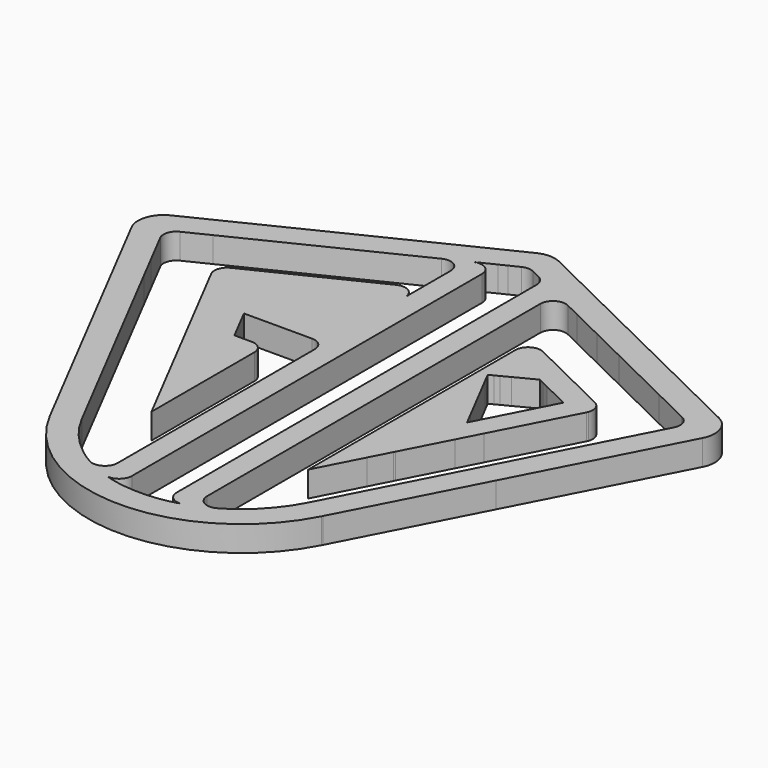
from build123d import *

# Parameters (mm, degrees)
F1_DEPTH = 1


# Not quite as in the source:
# - ends of sketch curves that miss each other by under 0.0002 mm in the source are joined
# - a feature names something its author has since deleted; it is built from what else it names


with BuildPart() as f1:
    # F0 (on Top) → F1 (new body)
    with BuildSketch(Plane.XY):
        with BuildLine():
            ThreePointArc((-11.7378467649, 8.9264858588), (-12.17732, 9.0282301738), (-12.6167932351, 8.9264858588))
            Line((-12.6167932351, 8.9264858588), (-22.9360292278, 3.8777807945))
            ThreePointArc((-22.9360292278, 3.8777807945), (-23.4460487393, 3.2933140895), (-23.3847383062, 2.5200338931))
            Line((-23.3847383062, 2.5200338931), (-17.5064138811, -8.8425854586))
            ThreePointArc((-17.5064138811, -8.8425854586), (-12.17732, -12.0856381601), (-6.8482261189, -8.8425854586))
            Line((-6.8482261189, -8.8425854586), (-6.8193229677, -8.786716561))
            Line((-6.8193229677, -8.786716561), (-4.1547760271, -3.6362297146))
            Line((-4.1547760271, -3.6362297146), (-0.9699016938, 2.5200338931))
            ThreePointArc((-0.9699016938, 2.5200338931), (-0.9085912607, 3.2933140895), (-1.4186107722, 3.8777807945))
            Line((-1.4186107722, 3.8777807945), (-11.7378467649, 8.9264858588))
        make_face()
        with BuildLine():
            ThreePointArc((-13.9352129405, -9.9781848161), (-14.1856518225, -10.4114506102), (-14.6860899339, -10.4106900001))
            ThreePointArc((-14.6860899339, -10.4106900001), (-14.9764347702, -10.2286994079), (-15.253632646, -10.0272495698))
            ThreePointArc((-15.253632646, -10.0272495698), (-16.0247836651, -9.2789159973), (-16.6182315676, -8.3830942422))
            Line((-16.6182315676, -8.3830942422), (-21.0987998739, 0.2777057515))
            Line((-21.0987998739, 0.2777057515), (-21.5773427489, 1.202714332))
            Line((-21.5773427489, 1.202714332), (-22.2616031934, 2.5253686134))
            ThreePointArc((-22.2616031934, 2.5253686134), (-22.29225841, 2.9120087116), (-22.0372486542, 3.2042420641))
            Line((-22.0372486542, 3.2042420641), (-21.0987998739, 3.6633798445))
            Line((-21.0987998739, 3.6633798445), (-14.6549495581, 6.8160453855))
            ThreePointArc((-14.6549495581, 6.8160453855), (-14.1705134022, 6.7911040048), (-13.9352129405, 6.366917543))
            Line((-13.9352129405, 6.366917543), (-13.9352129405, 4.1403800065))
            ThreePointArc((-13.9352129405, 4.1403800065), (-14.1705134022, 4.5645664683), (-14.6549495581, 4.589507849))
            Line((-14.6549495581, 4.589507849), (-15.253632646, 4.2966010544))
            Line((-15.253632646, 4.2966010544), (-18.9906600384, 2.4682535744))
            Line((-18.9906600384, 2.4682535744), (-18.5866887981, 1.687389658))
            Line((-18.5866887981, 1.687389658), (-16.9010777379, 2.5120779491))
            Line((-16.9010777379, 2.5120779491), (-14.6549495581, 3.6110002651))
            ThreePointArc((-14.6549495581, 3.6110002651), (-14.1705134022, 3.5860588844), (-13.9352129405, 3.1618724226))
            Line((-13.9352129405, 3.1618724226), (-13.9352129405, 1.0737917123))
            Line((-13.9352129405, 1.0737917123), (-13.9352129405, -0.3051582877))
            Line((-13.9352129405, -0.3051582877), (-13.9352129405, -9.9781848161))
        make_face(mode=Mode.SUBTRACT)
        with BuildLine():
            Line((-10.6659804544, -10.8341303593), (-10.4194270595, -10.7664300173))
            ThreePointArc((-10.4194270595, -10.7664300173), (-10.5663720437, -10.8190139832), (-10.7148866003, -10.8669861449))
            ThreePointArc((-10.7148866003, -10.8669861449), (-11.0045154737, -10.9461452883), (-11.2983735297, -11.0077772381))
            ThreePointArc((-11.2983735297, -11.0077772381), (-11.423285282, -11.0284543254), (-11.548680536, -11.0459619827))
            ThreePointArc((-11.548680536, -11.0459619827), (-11.6318465406, -11.0842260567), (-11.720595012, -11.1066856319))
            ThreePointArc((-11.720595012, -11.1066856319), (-12.17732, -11.1424265632), (-12.634044988, -11.1066856319))
            ThreePointArc((-12.634044988, -11.1066856319), (-12.7227934594, -11.0842260567), (-12.805959464, -11.0459619827))
            ThreePointArc((-12.805959464, -11.0459619827), (-12.931354718, -11.0284543254), (-13.0562664703, -11.0077772381))
            ThreePointArc((-13.0562664703, -11.0077772381), (-13.3501245263, -10.9461452883), (-13.6397533997, -10.8669861449))
            ThreePointArc((-13.6397533997, -10.8669861449), (-13.2335773511, -10.7559370641), (-13.0562664703, -10.3740054834))
            Line((-13.0562664703, -10.3740054834), (-13.0562664703, -10.0437429667))
            Line((-13.0562664703, -10.0437429667), (-13.0562664703, 5.3716664708))
            Line((-13.0562664703, 5.3716664708), (-13.0562664703, 6.7969437096))
            ThreePointArc((-13.0562664703, 6.7969437096), (-13.2915669319, 7.2211301714), (-13.7760030878, 7.246071552))
            Line((-13.7760030878, 7.246071552), (-13.0562664703, 7.5982040073))
            Line((-13.0562664703, 7.5982040073), (-12.7760030878, 7.7353233792))
            Line((-12.7760030878, 7.7353233792), (-12.3970566176, 7.9207236322))
            ThreePointArc((-12.3970566176, 7.9207236322), (-12.17732, 7.9715957897), (-11.9575833824, 7.9207236322))
            Line((-11.9575833824, 7.9207236322), (-11.5786369122, 7.7353233792))
            ThreePointArc((-11.5786369122, 7.7353233792), (-11.3741870679, 7.5508950751), (-11.2983735297, 7.2861955367))
            Line((-11.2983735297, 7.2861955367), (-11.2983735297, -10.0437429667))
            Line((-11.2983735297, -10.0437429667), (-11.2983735297, -10.3519767804))
            ThreePointArc((-11.2983735297, -10.3519767804), (-11.1015265128, -10.7495925105), (-10.6659804544, -10.8341303593))
        make_face(mode=Mode.SUBTRACT)
        with BuildLine():
            Line((-5.5053601225, -4.0705468447), (-6.0704119356, -5.1627745276))
            Line((-6.0704119356, -5.1627745276), (-6.8376335928, -6.6457902679))
            Line((-6.8376335928, -6.6457902679), (-7.7364084324, -8.3830942422))
            ThreePointArc((-7.7364084324, -8.3830942422), (-8.3298563349, -9.2789159973), (-9.101007354, -10.0272495698))
            ThreePointArc((-9.101007354, -10.0272495698), (-9.3782052298, -10.2286994079), (-9.6685500661, -10.4106900001))
            ThreePointArc((-9.6685500661, -10.4106900001), (-10.1689881775, -10.4114506102), (-10.4194270595, -9.9781848161))
            Line((-10.4194270595, -9.9781848161), (-10.4194270595, -1.8278266693))
            Line((-10.4194270595, -1.8278266693), (-10.4194270595, -0.3051582877))
            Line((-10.4194270595, -0.3051582877), (-10.4194270595, 0.2777057515))
            Line((-10.4194270595, 0.2777057515), (-10.4194270595, 0.5210568374))
            Line((-10.4194270595, 0.5210568374), (-10.4194270595, 3.0275448634))
            Line((-10.4194270595, 3.0275448634), (-10.4194270595, 4.6300693884))
            Line((-10.4194270595, 4.6300693884), (-10.4194270595, 6.366917543))
            Line((-10.4194270595, 6.366917543), (-10.4194270595, 7.1681778407))
            Line((-10.4194270595, 7.1681778407), (-9.6996904419, 6.8160453855))
            Line((-9.6996904419, 6.8160453855), (-9.101007354, 6.5231385909))
            Line((-9.101007354, 6.5231385909), (-7.825559943, 5.8991236145))
            Line((-7.825559943, 5.8991236145), (-6.386082692, 5.1948567393))
            Line((-6.386082692, 5.1948567393), (-3.816366891, 3.9376185884))
            Line((-3.816366891, 3.9376185884), (-2.3768901261, 3.2333519511))
            Line((-2.3768901261, 3.2333519511), (-2.3173913458, 3.2042420641))
            ThreePointArc((-2.3173913458, 3.2042420641), (-2.06238159, 2.9120087116), (-2.0930368066, 2.5253686134))
            Line((-2.0930368066, 2.5253686134), (-2.3768901261, 1.9766889238))
            Line((-2.3768901261, 1.9766889238), (-2.7772972511, 1.202714332))
            Line((-2.7772972511, 1.202714332), (-3.2558401261, 0.2777057515))
            Line((-3.2558401261, 0.2777057515), (-3.3676578126, 0.061565621))
            Line((-3.3676578126, 0.061565621), (-5.0612689658, -3.2121323703))
            Line((-5.0612689658, -3.2121323703), (-5.5053601225, -4.0705468447))
        make_face(mode=Mode.SUBTRACT)
        with BuildLine():
            Line((-16.5720523514, -4.1197169088), (-15.2536327446, -6.6681812422))
            Line((-15.2536327446, -6.6681812422), (-15.2536328928, -1.623578273))
            ThreePointArc((-15.2536328928, -1.623578273), (-15.4000795074, -1.2700248919), (-15.7536328928, -1.1235782877))
            Line((-15.7536328928, -1.1235782877), (-16.0720525039, -1.1235782877))
            Line((-16.0720525039, -1.1235782877), (-16.4336040792, -1.1235782877))
            Line((-16.4336040792, -1.1235782877), (-17.1154396337, 0.1948417123))
            Line((-17.1154396337, 0.1948417123), (-16.0720524345, 0.1948417123))
            Line((-16.0720524345, 0.1948417123), (-15.2536329075, 0.1948417123))
            Line((-15.2536329075, 0.1948417123), (-14.4352129405, 0.1948417123))
            ThreePointArc((-14.4352129405, 0.1948417123), (-14.08165955, 0.0483951029), (-13.9352129405, -0.3051582877))
            Line((-13.9352129405, -0.3051582877), (-13.9352129405, 1.0737917123))
            Line((-13.9352129405, 1.0737917123), (-15.2536329075, 1.0737917123))
            Line((-15.2536329075, 1.0737917123), (-18.2692507427, 1.0737917123))
            Line((-18.2692507427, 1.0737917123), (-18.6097401643, 1.0737917123))
            Line((-18.6097401643, 1.0737917123), (-19.1218068604, 0.8088797168))
            Line((-19.1218068604, 0.8088797168), (-16.5720523514, -4.1197169088))
        make_face()
        Polygon((-16.1325828631, -3.0563212317), (-16.6777508926, -2.0025282877), (-16.1325828631, -2.0025282877), (-16.1325828631, -2.6348403451), align=None, mode=Mode.SUBTRACT)
        with BuildLine():
            Line((-15.2536329075, 1.0737917123), (-13.9352129405, 1.0737917123))
            Line((-13.9352129405, 1.0737917123), (-13.9352129405, 3.1618724226))
            ThreePointArc((-13.9352129405, 3.1618724226), (-14.1705134022, 3.5860588844), (-14.6549495581, 3.6110002651))
            Line((-14.6549495581, 3.6110002651), (-16.9010777379, 2.5120779491))
            Line((-16.9010777379, 2.5120779491), (-18.5866887981, 1.687389658))
            Line((-18.5866887981, 1.687389658), (-18.3411390159, 1.2127495215))
            Line((-18.3411390159, 1.2127495215), (-18.2692507427, 1.0737917123))
            Line((-18.2692507427, 1.0737917123), (-15.2536329075, 1.0737917123))
        make_face()
        with BuildLine():
            Line((-19.5454273692, 1.6277250617), (-19.3764089282, 1.3010176414))
            Line((-19.3764089282, 1.3010176414), (-18.5866887981, 1.687389658))
            Line((-18.5866887981, 1.687389658), (-18.9906600384, 2.4682535744))
            Line((-18.9906600384, 2.4682535744), (-19.32107283, 2.3065985124))
            ThreePointArc((-19.32107283, 2.3065985124), (-19.5760825858, 2.01436516), (-19.5454273692, 1.6277250617))
        make_face()
        Polygon((-19.3764089282, 1.3010176414), (-19.1218068604, 0.8088797168), (-18.6097401643, 1.0737917123), (-18.3411390159, 1.2127495215), (-18.5866887981, 1.687389658), align=None)
        Polygon((-16.1325828631, -2.0025282877), (-16.6777508926, -2.0025282877), (-16.1325828631, -3.0563212317), (-16.1325828631, -2.6348403451), align=None)
        with BuildLine():
            Line((-10.4194270595, 7.1681778407), (-10.4194270595, 6.366917543))
            ThreePointArc((-10.4194270595, 6.366917543), (-10.1841265978, 6.7911040048), (-9.6996904419, 6.8160453855))
            Line((-9.6996904419, 6.8160453855), (-10.4194270595, 7.1681778407))
        make_face()
        with BuildLine():
            ThreePointArc((-11.720595012, -11.1066856319), (-11.6318465406, -11.0842260567), (-11.548680536, -11.0459619827))
            ThreePointArc((-11.548680536, -11.0459619827), (-12.17732, -11.0856381601), (-12.805959464, -11.0459619827))
            ThreePointArc((-12.805959464, -11.0459619827), (-12.7227934594, -11.0842260567), (-12.634044988, -11.1066856319))
            ThreePointArc((-12.634044988, -11.1066856319), (-12.17732, -11.1424265632), (-11.720595012, -11.1066856319))
        make_face()
        Polygon((-18.3411390159, 1.2127495215), (-18.6097401643, 1.0737917123), (-18.2692507427, 1.0737917123), align=None)
        with BuildLine():
            ThreePointArc((-10.7148866003, -10.8669861449), (-10.5663720437, -10.8190139832), (-10.4194270595, -10.7664300173))
            Line((-10.4194270595, -10.7664300173), (-10.6659804544, -10.8341303593))
            ThreePointArc((-10.6659804544, -10.8341303593), (-11.1015265128, -10.7495925105), (-11.2983735297, -10.3519767804))
            Line((-11.2983735297, -10.3519767804), (-11.2983735297, -10.3740054834))
            ThreePointArc((-11.2983735297, -10.3740054834), (-11.1210626489, -10.7559370641), (-10.7148866003, -10.8669861449))
        make_face()
    extrude(amount=F1_DEPTH)


with BuildPart() as f1b:
    # F0 (on Top) → F1, piece 2 (new body)
    with BuildSketch(Plane.XY):
        with BuildLine():
            Line((-9.1010072554, -6.6681812422), (-8.1977966169, -4.9223030059))
            ThreePointArc((-8.1977966169, -4.9223030059), (-8.6841611224, -4.6077302475), (-9.1010072685, -4.2055539889))
            Line((-9.1010072685, -4.2055539889), (-9.1010072554, -6.6681812422))
        make_face()
        with BuildLine():
            ThreePointArc((-9.1010072685, -4.2055539889), (-8.6841611224, -4.6077302475), (-8.1977966169, -4.9223030059))
            Line((-8.1977966169, -4.9223030059), (-7.7825876486, -4.1197169088))
            Line((-7.7825876486, -4.1197169088), (-7.7566160256, -4.0695145646))
            ThreePointArc((-7.7566160256, -4.0695145646), (-8.2518471552, -3.7073634999), (-8.6139982198, -3.2121323703))
            Line((-8.6139982198, -3.2121323703), (-9.101007354, -2.2707587726))
            Line((-9.101007354, -2.2707587726), (-9.101007354, -4.2055539889))
        make_face()
        with BuildLine():
            Line((-9.101007354, -1.623578273), (-9.101007354, -2.2707587726))
            Line((-9.101007354, -2.2707587726), (-8.6139982198, -3.2121323703))
            ThreePointArc((-8.6139982198, -3.2121323703), (-8.2518471552, -3.7073634999), (-7.7566160256, -4.0695145646))
            Line((-7.7566160256, -4.0695145646), (-6.8376335928, -2.2931499375))
            Line((-6.8376335928, -2.2931499375), (-6.393542436, -1.4347354631))
            ThreePointArc((-6.393542436, -1.4347354631), (-6.8376335928, -1.7049898549), (-7.2817247495, -1.4347354631))
            Line((-7.2817247495, -1.4347354631), (-8.8660545548, 1.6277250617))
            ThreePointArc((-8.8660545548, 1.6277250617), (-8.8784767188, 1.6535207057), (-8.8894020206, 1.6799850815))
            Line((-8.8894020206, 1.6799850815), (-9.101007354, 1.6799850815))
            Line((-9.101007354, 1.6799850815), (-9.101007354, -1.623578273))
        make_face()
        with BuildLine():
            Line((-9.101007354, 3.4953407566), (-9.101007354, 1.6799850815))
            Line((-9.101007354, 1.6799850815), (-8.8894020206, 1.6799850815))
            ThreePointArc((-8.8894020206, 1.6799850815), (-8.8869510867, 2.0412815765), (-8.6417000156, 2.3065985124))
            Line((-8.6417000156, 2.3065985124), (-7.2771068279, 2.9742282228))
            ThreePointArc((-7.2771068279, 2.9742282228), (-7.063182163, 3.0502044622), (-6.8376335928, 3.0759725378))
            Line((-6.8376335928, 3.0759725378), (-6.8376335928, 3.1892413061))
            Line((-6.8376335928, 3.1892413061), (-8.3812707365, 3.9444685991))
            ThreePointArc((-8.3812707365, 3.9444685991), (-8.8657068924, 3.9195272185), (-9.101007354, 3.4953407566))
        make_face()
        with BuildLine():
            ThreePointArc((-7.2817247495, -1.4347354631), (-6.8376335928, -1.7049898549), (-6.393542436, -1.4347354631))
            Line((-6.393542436, -1.4347354631), (-4.8092126308, 1.6277250617))
            ThreePointArc((-4.8092126308, 1.6277250617), (-4.7951941207, 1.6571321237), (-4.7831203666, 1.687389658))
            Line((-4.7831203666, 1.687389658), (-5.7679512019, 1.687389658))
            Line((-5.7679512019, 1.687389658), (-6.8376335928, -0.3802733283))
            Line((-6.8376335928, -0.3802733283), (-6.9415896155, -0.5812171058))
            Line((-6.9415896155, -0.5812171058), (-7.0455456382, -0.7821608834))
            Line((-7.0455456382, -0.7821608834), (-7.0456700866, -0.7824014383))
            Line((-7.0456700866, -0.7824014383), (-7.1495016609, -0.9831046609))
            Line((-7.1495016609, -0.9831046609), (-7.2534576837, -1.1840484384))
            Line((-7.2534576837, -1.1840484384), (-7.4936940826, -0.7196789075))
            Line((-7.4936940826, -0.7196789075), (-8.5595457985, 1.3405795023))
            Line((-8.5595457985, 1.3405795023), (-8.6542783092, 1.5236945164))
            Line((-8.6542783092, 1.5236945164), (-8.6912365674, 1.5951336867))
            Line((-8.6912365674, 1.5951336867), (-8.7351334904, 1.6799850815))
            Line((-8.7351334904, 1.6799850815), (-8.8894020206, 1.6799850815))
            ThreePointArc((-8.8894020206, 1.6799850815), (-8.8784767188, 1.6535207057), (-8.8660545548, 1.6277250617))
            Line((-8.8660545548, 1.6277250617), (-7.2817247495, -1.4347354631))
        make_face()
        with BuildLine():
            ThreePointArc((-8.6417000156, 2.3065985124), (-8.8869510867, 2.0412815765), (-8.8894020206, 1.6799850815))
            Line((-8.8894020206, 1.6799850815), (-8.7351334904, 1.6799850815))
            Line((-8.7351334904, 1.6799850815), (-8.5654128233, 1.7677881761))
            Line((-8.5654128233, 1.7677881761), (-8.3994958527, 1.8536234709))
            Line((-8.3994958527, 1.8536234709), (-8.0790730005, 2.0193906606))
            Line((-8.0790730005, 2.0193906606), (-7.285583076, 2.4298938254))
            Line((-7.285583076, 2.4298938254), (-7.1787263557, 2.3776139797))
            Line((-7.1787263557, 2.3776139797), (-6.8376335928, 2.5540745174))
            Line((-6.8376335928, 2.5540745174), (-6.8376335928, 3.0759725378))
            ThreePointArc((-6.8376335928, 3.0759725378), (-7.063182163, 3.0502044622), (-7.2771068279, 2.9742282228))
            Line((-7.2771068279, 2.9742282228), (-8.6417000156, 2.3065985124))
        make_face()
        with BuildLine():
            Line((-5.7679512019, 1.687389658), (-4.7831203666, 1.687389658))
            ThreePointArc((-4.7831203666, 1.687389658), (-4.7897821416, 2.0449478252), (-5.03356717, 2.3065985124))
            Line((-5.03356717, 2.3065985124), (-6.3981603577, 2.9742282228))
            ThreePointArc((-6.3981603577, 2.9742282228), (-6.6120850226, 3.0502044622), (-6.8376335928, 3.0759725378))
            Line((-6.8376335928, 3.0759725378), (-6.8376335928, 2.5540745174))
            Line((-6.8376335928, 2.5540745174), (-6.8376335928, 2.3389525605))
            Line((-6.8376335928, 2.3389525605), (-6.8376335928, 2.2107337222))
            Line((-6.8376335928, 2.2107337222), (-5.7679512019, 1.687389658))
        make_face()
        with BuildLine():
            Line((-6.3981603577, 2.9742282228), (-6.8376335928, 3.1892413061))
            Line((-6.8376335928, 3.1892413061), (-6.8376335928, 3.0759725378))
            ThreePointArc((-6.8376335928, 3.0759725378), (-6.6120850226, 3.0502044622), (-6.3981603577, 2.9742282228))
        make_face()
        Polygon((-6.8581561948, 2.2207744428), (-6.8376335928, 2.2107337222), (-6.8376335928, 2.3389525605), (-6.9650129151, 2.2730542884), align=None)
        Polygon((-6.8376335928, 2.3389525605), (-6.8376335928, 2.5540745174), (-7.1787263557, 2.3776139797), (-7.1601386162, 2.3685198942), (-7.0718696354, 2.3253341341), (-7.0648745265, 2.3219117643), (-6.9650129151, 2.2730542884), align=None)
    extrude(amount=F1_DEPTH)


solid = Compound([f1.part, f1b.part])
